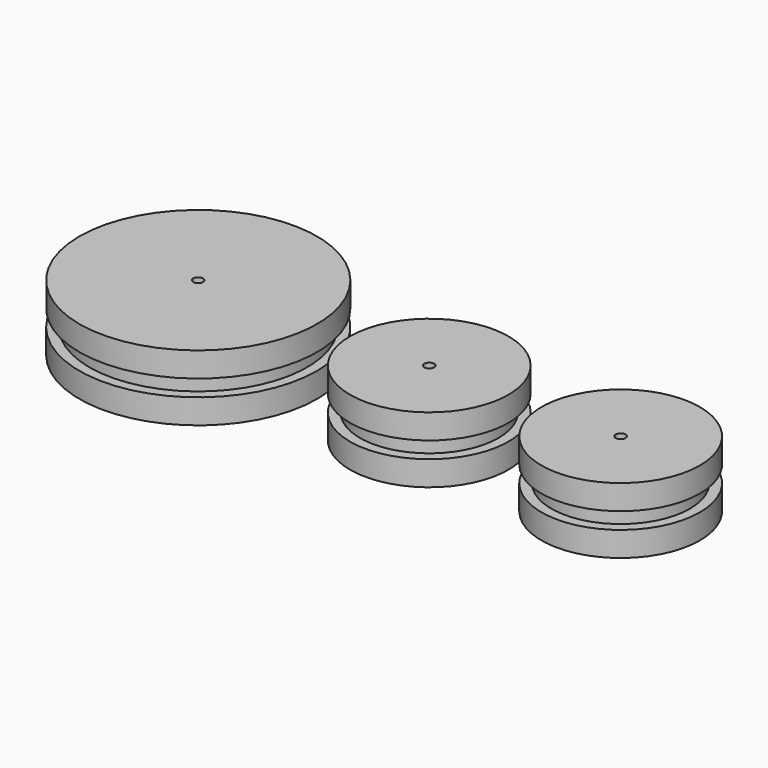
from build123d import *

# Parameters (mm, degrees)
F1_DEPTH = 7.5
F2_DEPTH = 12.5
F3_START = 12.5
F3_DEPTH = 7.5
F5_DEPTH = 7.5
F4_R     = 24
F4_R_2   = 21
F4_R_3   = 1.5
F6_DEPTH = 12.5
F7_START = 12.5
F7_DEPTH = 7.5


with BuildPart() as f1:
    # F0 (on Top) → F1 (new body)
    with BuildSketch(Plane.XY):
        with BuildLine():
            Line((21, 0), (24, 0))
            ThreePointArc((24, 0), (0, 24), (-24, 0))
            Line((-24, 0), (-21, 0))
            ThreePointArc((-21, 0), (0, 21), (21, 0))
        make_face()
        with BuildLine():
            ThreePointArc((-24, 0), (0, -24), (24, 0))
            Line((24, 0), (21, 0))
            ThreePointArc((21, 0), (0, -21), (-21, 0))
            Line((-21, 0), (-24, 0))
        make_face()
        with BuildLine():
            ThreePointArc((-21, 0), (0, -21), (21, 0))
            Line((21, 0), (1.5, 0))
            ThreePointArc((1.5, 0), (0, -1.5), (-1.5, 0))
            Line((-1.5, 0), (-21, 0))
        make_face()
        with BuildLine():
            Line((1.5, 0), (21, 0))
            ThreePointArc((21, 0), (0, 21), (-21, 0))
            Line((-21, 0), (-1.5, 0))
            ThreePointArc((-1.5, 0), (0, 1.5), (1.5, 0))
        make_face()
    extrude(amount=F1_DEPTH)

    # F0 (on Top) → F2 (join)
    with BuildSketch(Plane.XY):
        with BuildLine():
            ThreePointArc((-21, 0), (0, -21), (21, 0))
            Line((21, 0), (1.5, 0))
            ThreePointArc((1.5, 0), (0, -1.5), (-1.5, 0))
            Line((-1.5, 0), (-21, 0))
        make_face()
        with BuildLine():
            Line((1.5, 0), (21, 0))
            ThreePointArc((21, 0), (0, 21), (-21, 0))
            Line((-21, 0), (-1.5, 0))
            ThreePointArc((-1.5, 0), (0, 1.5), (1.5, 0))
        make_face()
    extrude(amount=F2_DEPTH)


with BuildPart() as f3:
    # F0 (on Top) → F3 (new body)
    with BuildSketch(Plane.XY.offset(F3_START)):
        with BuildLine():
            Line((21, 0), (24, 0))
            ThreePointArc((24, 0), (0, 24), (-24, 0))
            Line((-24, 0), (-21, 0))
            ThreePointArc((-21, 0), (0, 21), (21, 0))
        make_face()
        with BuildLine():
            ThreePointArc((-24, 0), (0, -24), (24, 0))
            Line((24, 0), (21, 0))
            ThreePointArc((21, 0), (0, -21), (-21, 0))
            Line((-21, 0), (-24, 0))
        make_face()
        with BuildLine():
            ThreePointArc((-21, 0), (0, -21), (21, 0))
            Line((21, 0), (1.5, 0))
            ThreePointArc((1.5, 0), (0, -1.5), (-1.5, 0))
            Line((-1.5, 0), (-21, 0))
        make_face()
        with BuildLine():
            Line((1.5, 0), (21, 0))
            ThreePointArc((21, 0), (0, 21), (-21, 0))
            Line((-21, 0), (-1.5, 0))
            ThreePointArc((-1.5, 0), (0, 1.5), (1.5, 0))
        make_face()
    extrude(amount=F3_DEPTH)


with BuildPart() as f5:
    # F4 (on Top) → F5 (new body)
    with BuildSketch(Plane.XY):
        with BuildLine():
            Line((-68.5, 0), (-37, 0))
            ThreePointArc((-37, 0), (-70, 33), (-103, 0))
            Line((-103, 0), (-71.5, 0))
            ThreePointArc((-71.5, 0), (-70, 1.5), (-68.5, 0))
        make_face()
        with BuildLine():
            ThreePointArc((-103, 0), (-70, -33), (-37, 0))
            Line((-37, 0), (-68.5, 0))
            ThreePointArc((-68.5, 0), (-70, -1.5), (-71.5, 0))
            Line((-71.5, 0), (-103, 0))
        make_face()
        with BuildLine():
            ThreePointArc((-106, 0), (-70, -36), (-34, 0))
            Line((-34, 0), (-37, 0))
            ThreePointArc((-37, 0), (-70, -33), (-103, 0))
            Line((-103, 0), (-106, 0))
        make_face()
        with BuildLine():
            Line((-37, 0), (-34, 0))
            ThreePointArc((-34, 0), (-70, 36), (-106, 0))
            Line((-106, 0), (-103, 0))
            ThreePointArc((-103, 0), (-70, 33), (-37, 0))
        make_face()
    extrude(amount=F5_DEPTH)


with BuildPart() as f5b:
    # F4 (on Top) → F5, piece 2 (new body)
    with BuildSketch(Plane.XY):
        with Locations((58, 0)):
            Circle(F4_R)
        with Locations((58, 0)):
            Circle(F4_R_2, mode=Mode.SUBTRACT)
        with Locations((58, 0)):
            Circle(F4_R_2)
        with Locations((58, 0)):
            Circle(F4_R_3, mode=Mode.SUBTRACT)
    extrude(amount=F5_DEPTH)


with BuildPart() as f6:
    # F4 (on Top) → F6 (new body)
    with BuildSketch(Plane.XY):
        with BuildLine():
            Line((-68.5, 0), (-37, 0))
            ThreePointArc((-37, 0), (-70, 33), (-103, 0))
            Line((-103, 0), (-71.5, 0))
            ThreePointArc((-71.5, 0), (-70, 1.5), (-68.5, 0))
        make_face()
        with BuildLine():
            ThreePointArc((-103, 0), (-70, -33), (-37, 0))
            Line((-37, 0), (-68.5, 0))
            ThreePointArc((-68.5, 0), (-70, -1.5), (-71.5, 0))
            Line((-71.5, 0), (-103, 0))
        make_face()
    extrude(amount=F6_DEPTH)


with BuildPart() as f6b:
    # F4 (on Top) → F6, piece 2 (new body)
    with BuildSketch(Plane.XY):
        with Locations((58, 0)):
            Circle(F4_R_2)
        with Locations((58, 0)):
            Circle(F4_R_3, mode=Mode.SUBTRACT)
    extrude(amount=F6_DEPTH)


with BuildPart() as f7:
    # F4 (on Top) → F7 (new body)
    with BuildSketch(Plane.XY.offset(F7_START)):
        with BuildLine():
            ThreePointArc((-103, 0), (-70, -33), (-37, 0))
            Line((-37, 0), (-68.5, 0))
            ThreePointArc((-68.5, 0), (-70, -1.5), (-71.5, 0))
            Line((-71.5, 0), (-103, 0))
        make_face()
        with BuildLine():
            Line((-68.5, 0), (-37, 0))
            ThreePointArc((-37, 0), (-70, 33), (-103, 0))
            Line((-103, 0), (-71.5, 0))
            ThreePointArc((-71.5, 0), (-70, 1.5), (-68.5, 0))
        make_face()
        with BuildLine():
            Line((-37, 0), (-34, 0))
            ThreePointArc((-34, 0), (-70, 36), (-106, 0))
            Line((-106, 0), (-103, 0))
            ThreePointArc((-103, 0), (-70, 33), (-37, 0))
        make_face()
        with BuildLine():
            ThreePointArc((-106, 0), (-70, -36), (-34, 0))
            Line((-34, 0), (-37, 0))
            ThreePointArc((-37, 0), (-70, -33), (-103, 0))
            Line((-103, 0), (-106, 0))
        make_face()
    extrude(amount=F7_DEPTH)


with BuildPart() as f7b:
    # F4 (on Top) → F7, piece 2 (new body)
    with BuildSketch(Plane.XY.offset(F7_START)):
        with Locations((58, 0)):
            Circle(F4_R)
        with Locations((58, 0)):
            Circle(F4_R_2, mode=Mode.SUBTRACT)
        with Locations((58, 0)):
            Circle(F4_R_2)
        with Locations((58, 0)):
            Circle(F4_R_3, mode=Mode.SUBTRACT)
    extrude(amount=F7_DEPTH)


solid = Compound([f1.part, f3.part, f5.part, f5b.part, f6.part, f6b.part, f7.part, f7b.part])
